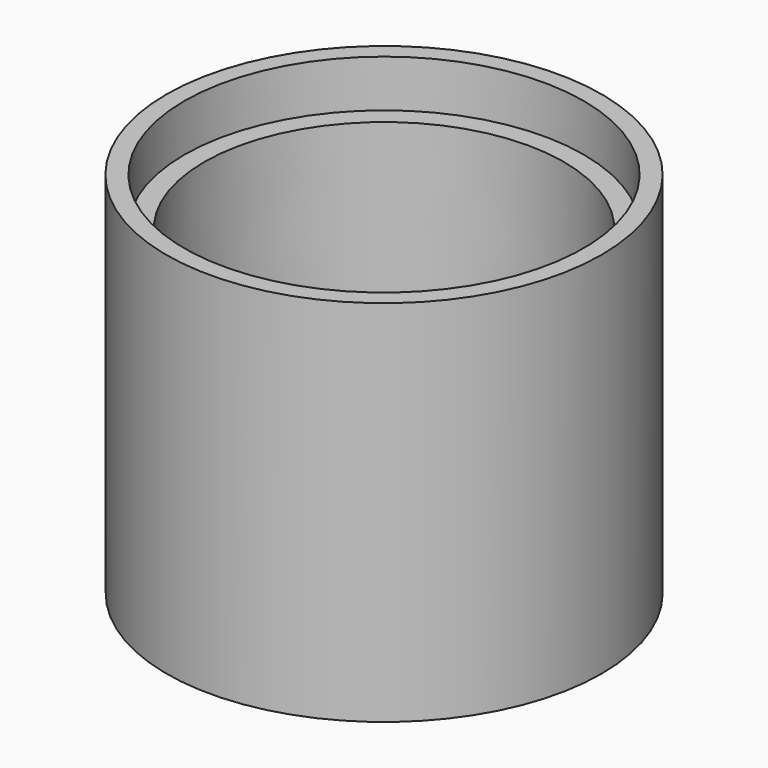
from build123d import *


with BuildPart() as f1:
    # F0 (on Front) → F1 (revolve)
    with BuildSketch(Plane.XZ):
        Polygon((-18.8000003844, 27.2467982708), (-20.8999994888, 27.244858796), (-20.8999994888, 32.2467982708), (-22.7999994888, 32.2467982708), (-22.7671931058, -6.7532017292), (0.2328019897, -6.7319598573), (0.2314215907, -3.7426586793), (-14.9668533656, -3.7426586793), (-14.9703099348, 0), (-18.7703107451, 0), align=None)
    revolve(axis=Axis((0.2321117902, 0, -5.2373092683), (0.0004617798, 0, -0.9999998934)))


solid = f1.part
